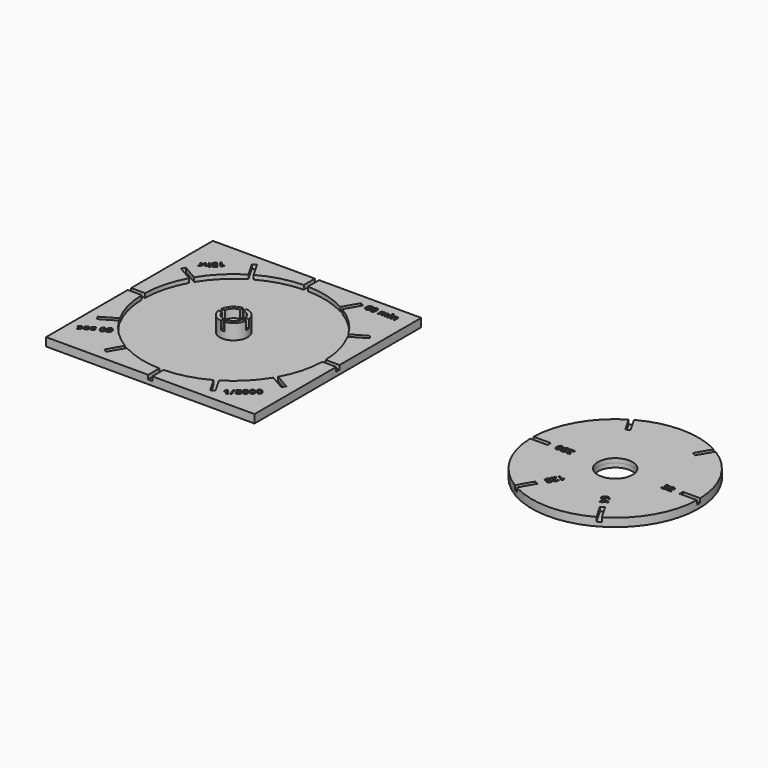
from build123d import *

# Parameters (mm, degrees)
F0_W          = 30
F0_H          = 30
F0_R          = 13
F0_R_2        = 2
F1_DEPTH      = 0.6
F0_R_3        = 12
F0_R_4        = 2.5
F2_DEPTH      = 0.6
F3_DEPTH      = 2.2
F3_DEPTH_BACK = 0.6
F4_W          = 0.5
F4_H          = 0.5
F5_DEPTH      = 1.2
F6_W          = 5
F6_H          = 0.6
F6_W_2        = 0.6
F6_H_2        = 5
F7_DEPTH      = 0.6
F8_W          = 5
F8_H          = 0.6
F9_DEPTH      = 0.6
F10_TEXT_SIZE = 1.3888888889
F11_DEPTH     = 0.6
F12_TEXT_SIZE = 1.3888888889
F13_DEPTH     = 0.6


# Not quite as in the source:
# - Text() gives the source's letters only with a copy of the font that has no kerning and outlines rounded to 1/6400 em; it was checked with that copy


with BuildPart() as f1:
    # F0 (on Top) → F1 (new body)
    with BuildSketch(Plane.XY):
        Rectangle(F0_W, F0_H)
        Circle(F0_R, mode=Mode.SUBTRACT)
        Circle(F0_R)
        Circle(F0_R_2, mode=Mode.SUBTRACT)
        Circle(F0_R_2)
    extrude(amount=-F1_DEPTH)

    # F0 (on Top) → F2 (join)
    with BuildSketch(Plane.XY):
        Rectangle(F0_W, F0_H)
        Circle(F0_R, mode=Mode.SUBTRACT)
    extrude(amount=F2_DEPTH)

    # F0 (on Top) → F3 (join, two sides)
    with BuildSketch(Plane.XY) as f3_sk:
        Circle(F0_R_2)
    extrude(amount=F3_DEPTH)
    extrude(f3_sk.sketch, amount=-F3_DEPTH_BACK)

    # F4 (on face) → F5 (cut)
    with BuildSketch(Plane.XY.offset(2.2)):
        with BuildLine():
            Line((5, -0.25), (5, 0.25))
            Line((5, 0.25), (1.4790199458, 0.25))
            ThreePointArc((1.4790199458, 0.25), (1.4947457842, 0.1254393904), (1.5, 0))
            ThreePointArc((1.5, 0), (1.4947457842, -0.1254393904), (1.4790199458, -0.25))
            Line((1.4790199458, -0.25), (5, -0.25))
        make_face()
        with BuildLine():
            ThreePointArc((1.5, 0), (1.4947457842, 0.1254393904), (1.4790199458, 0.25))
            Line((1.4790199458, 0.25), (0.25, 0.25))
            Line((0.25, 0.25), (0.25, -0.25))
            Line((0.25, -0.25), (1.4790199458, -0.25))
            ThreePointArc((1.4790199458, -0.25), (1.4947457842, -0.1254393904), (1.5, 0))
        make_face()
        with BuildLine():
            Line((0.25, 0.25), (1.4790199458, 0.25))
            ThreePointArc((1.4790199458, 0.25), (1.0606601718, 1.0606601718), (0.25, 1.4790199458))
            Line((0.25, 1.4790199458), (0.25, 0.25))
        make_face()
        with BuildLine():
            Line((-0.25, 0.25), (0.25, 0.25))
            Line((0.25, 0.25), (0.25, 1.4790199458))
            ThreePointArc((0.25, 1.4790199458), (0, 1.5), (-0.25, 1.4790199458))
            Line((-0.25, 1.4790199458), (-0.25, 0.25))
        make_face()
        with BuildLine():
            ThreePointArc((-0.25, 1.4790199458), (0, 1.5), (0.25, 1.4790199458))
            Line((0.25, 1.4790199458), (0.25, 5))
            Line((0.25, 5), (-0.25, 5))
            Line((-0.25, 5), (-0.25, 1.4790199458))
        make_face()
        with BuildLine():
            ThreePointArc((0.25, -1.4790199458), (1.0606601718, -1.0606601718), (1.4790199458, -0.25))
            Line((1.4790199458, -0.25), (0.25, -0.25))
            Line((0.25, -0.25), (0.25, -1.4790199458))
        make_face()
        with BuildLine():
            Line((-0.25, -0.25), (-0.25, 0.25))
            Line((-0.25, 0.25), (-1.4790199458, 0.25))
            ThreePointArc((-1.4790199458, 0.25), (-1.5, 0), (-1.4790199458, -0.25))
            Line((-1.4790199458, -0.25), (-0.25, -0.25))
        make_face()
        with BuildLine():
            Line((-1.4790199458, 0.25), (-0.25, 0.25))
            Line((-0.25, 0.25), (-0.25, 1.4790199458))
            ThreePointArc((-0.25, 1.4790199458), (-1.0606601718, 1.0606601718), (-1.4790199458, 0.25))
        make_face()
        with BuildLine():
            Line((0.25, -1.4790199458), (0.25, -0.25))
            Line((0.25, -0.25), (-0.25, -0.25))
            Line((-0.25, -0.25), (-0.25, -1.4790199458))
            ThreePointArc((-0.25, -1.4790199458), (0, -1.5), (0.25, -1.4790199458))
        make_face()
        with BuildLine():
            Line((0.25, -5), (0.25, -1.4790199458))
            ThreePointArc((0.25, -1.4790199458), (0, -1.5), (-0.25, -1.4790199458))
            Line((-0.25, -1.4790199458), (-0.25, -5))
            Line((-0.25, -5), (0.25, -5))
        make_face()
        with BuildLine():
            ThreePointArc((-1.4790199458, -0.25), (-1.5, 0), (-1.4790199458, 0.25))
            Line((-1.4790199458, 0.25), (-5, 0.25))
            Line((-5, 0.25), (-5, -0.25))
            Line((-5, -0.25), (-1.4790199458, -0.25))
        make_face()
        with BuildLine():
            Line((-0.25, -1.4790199458), (-0.25, -0.25))
            Line((-0.25, -0.25), (-1.4790199458, -0.25))
            ThreePointArc((-1.4790199458, -0.25), (-1.0606601718, -1.0606601718), (-0.25, -1.4790199458))
        make_face()
        Rectangle(F4_W, F4_H)
    extrude(amount=-F5_DEPTH, mode=Mode.SUBTRACT)

    # F6 (on face) → F7 (cut, through all)
    with BuildSketch(Plane.XY.offset(0.6)):
        with Locations((13, 0)):
            Rectangle(F6_W, F6_H)
        Polygon((8.9432667397, 5.5098076211), (9.2432667397, 4.9901923789), (13.5733937587, 7.4901923789), (13.2733937587, 8.0098076211), align=None)
        Polygon((4.9901923789, 9.2432667397), (5.5098076211, 8.9432667397), (8.0098076211, 13.2733937587), (7.4901923789, 13.5733937587), align=None)
        with Locations((0, 13)):
            Rectangle(F6_W_2, F6_H_2)
        Polygon((-5.5098076211, 8.9432667397), (-4.9901923789, 9.2432667397), (-7.4901923789, 13.5733937587), (-8.0098076211, 13.2733937587), align=None)
        Polygon((-9.2432667397, 4.9901923789), (-8.9432667397, 5.5098076211), (-13.2733937587, 8.0098076211), (-13.5733937587, 7.4901923789), align=None)
        with Locations((-13, 0)):
            Rectangle(F6_W, F6_H)
        Polygon((-8.9432667397, -5.5098076211), (-9.2432667397, -4.9901923789), (-13.5733937587, -7.4901923789), (-13.2733937587, -8.0098076211), align=None)
        Polygon((-4.9901923789, -9.2432667397), (-5.5098076211, -8.9432667397), (-8.0098076211, -13.2733937587), (-7.4901923789, -13.5733937587), align=None)
        with Locations((0, -13)):
            Rectangle(F6_W_2, F6_H_2)
        Polygon((5.5098076211, -8.9432667397), (4.9901923789, -9.2432667397), (7.4901923789, -13.5733937587), (8.0098076211, -13.2733937587), align=None)
        Polygon((9.2432667397, -4.9901923789), (8.9432667397, -5.5098076211), (13.2733937587, -8.0098076211), (13.5733937587, -7.4901923789), align=None)
    extrude(amount=-F7_DEPTH, mode=Mode.SUBTRACT)

    # F12 (on face) → F13 (cut, through all)
    with BuildSketch(Plane.XY.offset(0.6)):
        with Locations((8.4751043675, 12.7061837985)):
            Text('60 min', F12_TEXT_SIZE, font='Open Sans', font_style=FontStyle.BOLD, text_align=(TextAlign.LEFT, TextAlign.BOTTOM))
        with Locations(Location((9.1879246202, -13.4223345272), (0, 0, 40))):
            Text('1/8000', F12_TEXT_SIZE, font='Open Sans', font_style=FontStyle.BOLD, text_align=(TextAlign.LEFT, TextAlign.BOTTOM))
        with Locations(Location((-10.3780456519, -8.5576738839), (0, 0, -150))):
            Text('60 sec', F12_TEXT_SIZE, font='Open Sans', font_style=FontStyle.BOLD, text_align=(TextAlign.LEFT, TextAlign.BOTTOM))
        with Locations(Location((-10.6050720192, 11.7378212105), (0, 0, -140))):
            Text('15hr', F12_TEXT_SIZE, font='Open Sans', font_style=FontStyle.BOLD, text_align=(TextAlign.LEFT, TextAlign.BOTTOM))
    extrude(amount=-F13_DEPTH, mode=Mode.SUBTRACT)


with BuildPart() as f1b:
    # F0 (on Top) → F1, piece 2 (new body)
    with BuildSketch(Plane.XY):
        with Locations((54.9200177193, 0)):
            Circle(F0_R_3)
        with Locations((54.9200177193, 0)):
            Circle(F0_R_4, mode=Mode.SUBTRACT)
    extrude(amount=-F1_DEPTH)

    # F0 (on Top) → F2, piece 2 (join)
    with BuildSketch(Plane.XY):
        with Locations((54.9200177193, 0)):
            Circle(F0_R_3)
        with Locations((54.9200177193, 0)):
            Circle(F0_R_4, mode=Mode.SUBTRACT)
    extrude(amount=F2_DEPTH)

    # F8 (on face) → F9 (cut)
    with BuildSketch(Plane.XY.offset(0.6)):
        with Locations((66.9200177193, 0)):
            Rectangle(F8_W, F8_H)
        Polygon((59.4102100981, 8.377241336), (59.9298253404, 8.077241336), (62.4298253404, 12.4073683549), (61.9102100981, 12.7073683549), align=None)
        Polygon((49.9102100981, 8.077241336), (50.4298253404, 8.377241336), (47.9298253404, 12.7073683549), (47.4102100981, 12.4073683549), align=None)
        with Locations((42.9200177193, 0)):
            Rectangle(F8_W, F8_H)
        Polygon((50.4298253404, -8.377241336), (49.9102100981, -8.077241336), (47.4102100981, -12.4073683549), (47.9298253404, -12.7073683549), align=None)
        Polygon((59.9298253404, -8.077241336), (59.4102100981, -8.377241336), (61.9102100981, -12.7073683549), (62.4298253404, -12.4073683549), align=None)
    extrude(amount=-F9_DEPTH, mode=Mode.SUBTRACT)

    # F10 (on face) → F11 (cut, through all)
    with BuildSketch(Plane.XY.offset(0.6)):
        with Locations((61.7885073026, -0.4947529014)):
            Text('32', F10_TEXT_SIZE, font='Open Sans', font_style=FontStyle.BOLD, text_align=(TextAlign.LEFT, TextAlign.BOTTOM))
        with Locations(Location((57.9100735938, -6.1789286921), (0, 0, -60))):
            Text('64', F10_TEXT_SIZE, font='Open Sans', font_style=FontStyle.BOLD, text_align=(TextAlign.LEFT, TextAlign.BOTTOM))
        with Locations(Location((51.4400215104, -5.0275302439), (0, 0, -120))):
            Text('125', F10_TEXT_SIZE, font='Open Sans', font_style=FontStyle.BOLD, text_align=(TextAlign.LEFT, TextAlign.BOTTOM))
        with Locations(Location((48.8388545248, 0.5), (0, 0, -180))):
            Text('250', F10_TEXT_SIZE, font='Open Sans', font_style=FontStyle.BOLD, text_align=(TextAlign.LEFT, TextAlign.BOTTOM))
    extrude(amount=-F11_DEPTH, mode=Mode.SUBTRACT)


solid = Compound([f1.part, f1b.part])
